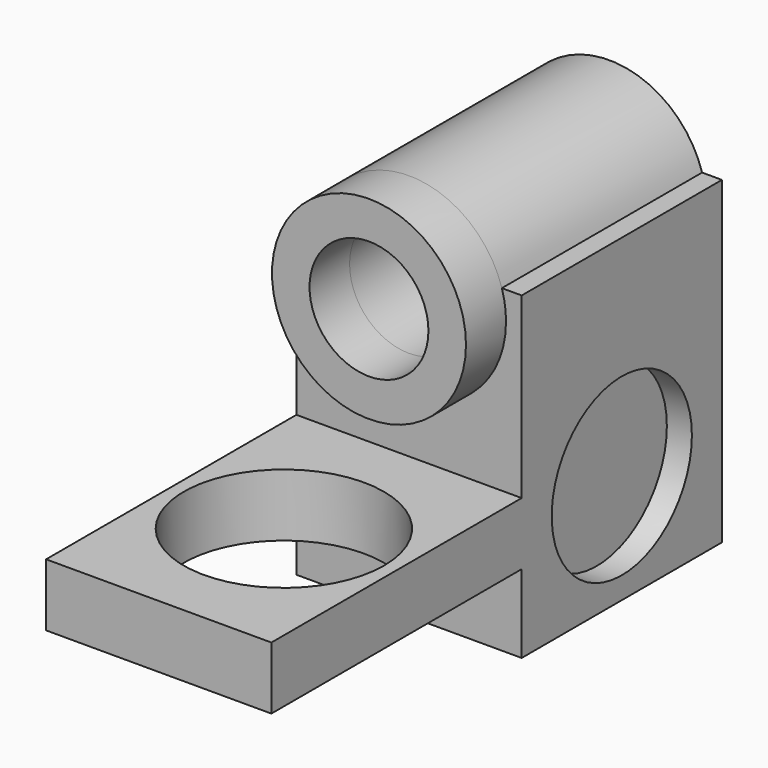
from build123d import *

# Parameters (mm, degrees)
F0_W          = 80
F0_H          = 102
F1_DEPTH      = 36
F2_W          = 100
F2_H          = 20
F3_DEPTH      = 72
F4_R          = 28
F5_DEPTH      = 8
F6_R          = 31
F6_R_2        = 19
F7_DEPTH      = 16
F7_DEPTH_BACK = 80
F8_DEPTH      = 80.001
F9_R          = 32
F10_DEPTH     = 45.001


# Not quite as in the source:
# - a pattern or mirror of a feature is missing from the dataset's text; its kind, count and spacing are read off the source's solid


with BuildPart() as f1:
    # F0 (on Right) → F1 (new body, symmetric)
    with BuildSketch(Plane.YZ):
        Rectangle(F0_W, F0_H)
    extrude(amount=F1_DEPTH, both=True)

    # F2 (on face) → F3 (join, through all)
    with BuildSketch(Plane.YZ.offset(36)):
        with Locations((-90, -16)):
            Rectangle(F2_W, F2_H)
    extrude(amount=-F3_DEPTH)

    # F4 (on face) → F5 (cut)
    with BuildSketch(Plane.YZ.offset(36)):
        with Locations((0, -16)):
            Circle(F4_R)
    f5 = extrude(amount=-F5_DEPTH, mode=Mode.SUBTRACT)

    # F5_copies: F5 across plane
    add(f5.mirror(Plane(origin=(0, 0, 0), x_dir=(0, 0, -1), z_dir=(-1, 0, 0))), mode=Mode.SUBTRACT)

    # F6 (on face) → F7 (join, two sides)
    with BuildSketch(Plane.XZ.offset(40)) as f7_sk:
        with Locations((0, 42)):
            Circle(F6_R)
        with Locations((0, 42)):
            Circle(F6_R_2, mode=Mode.SUBTRACT)
    extrude(amount=F7_DEPTH)
    extrude(f7_sk.sketch, amount=-F7_DEPTH_BACK)

    # F8 (cut, through all): a face of the model
    f8_faces = [f1.faces().sort_by_distance(p)[0] for p in [
        (0, -40, 38.5131332961),
    ]]
    extrude(f8_faces, amount=-F8_DEPTH, mode=Mode.SUBTRACT)

    # F9 (on face) → F10 (cut, through all)
    with BuildSketch(Plane.XY.offset(-6)):
        with Locations((0, -90)):
            Circle(F9_R)
    extrude(amount=-F10_DEPTH, mode=Mode.SUBTRACT)


solid = f1.part
